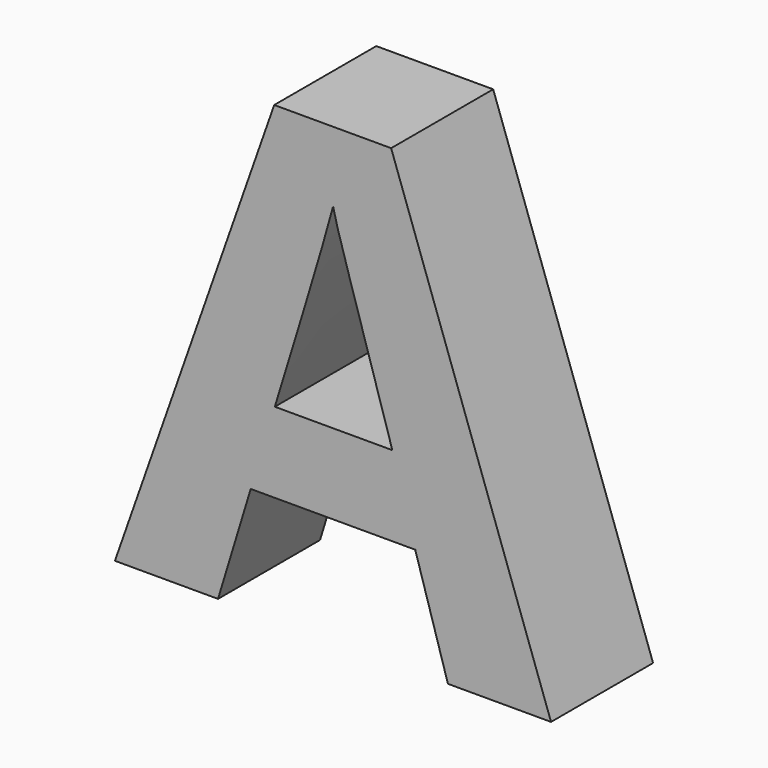
from build123d import *

# Parameters (mm, degrees)
F0_TEXT_SIZE = 125.8592793925
F1_DEPTH     = 25.4


# Not quite as in the source:
# - Text() gives the source's letters only with a copy of the font that has no kerning and outlines rounded to 1/6400 em; it was checked with that copy


with BuildPart() as f1:
    # F0 (on Front) → F1 (new body)
    with BuildSketch(Plane.XZ):
        with Locations((-57.9028762877, -42.8453870118)):
            Text('A', F0_TEXT_SIZE, font='Open Sans', font_style=FontStyle.BOLD, text_align=(TextAlign.LEFT, TextAlign.BOTTOM))
    extrude(amount=F1_DEPTH)


solid = f1.part
